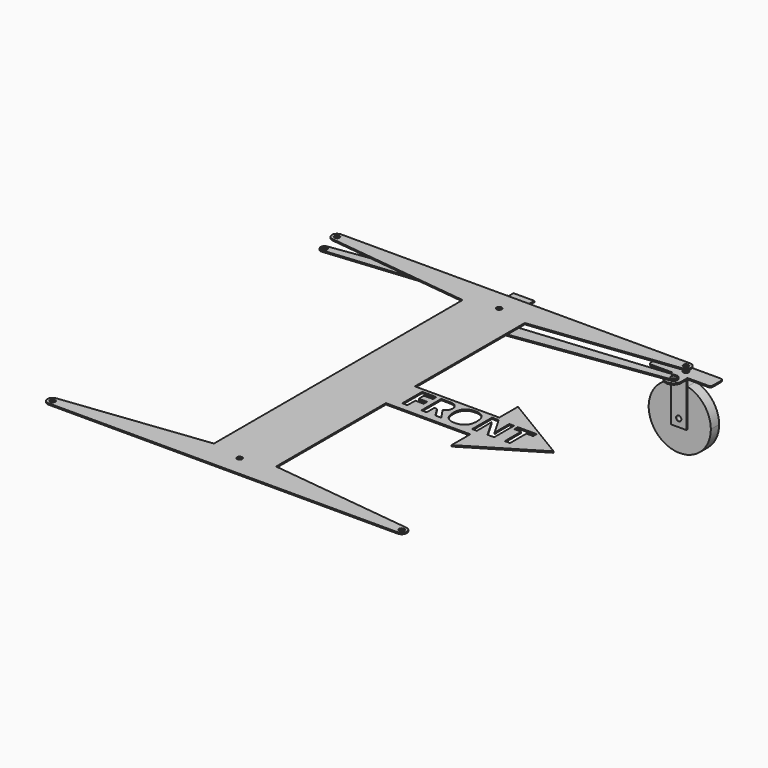
from build123d import *

# Parameters (mm, degrees)
F0_R      = 6.35
F1_DEPTH  = 3.175
F2_DEPTH  = 3.175
F3_R      = 6.35
F4_DEPTH  = 3.175
F6_R      = 6.35
F7_DEPTH  = 3.175
F8_R      = 6.35
F9_DEPTH  = 3.175
F10_DEPTH = 25.4


# Not quite as in the source:
# - a feature names something its author has since deleted; it is built from what else it names


with BuildPart() as f1:
    # F0 (on Top) → F1 (new body)
    with BuildSketch(Plane.XY):
        with BuildLine():
            Line((25.4, -29.2133073411), (25.4, 76.2))
            Line((25.4, 76.2), (-25.4, 76.2))
            Line((-25.4, 76.2), (-25.4, 66.4512439966))
            Line((-25.4, 66.4512439966), (-2.6644509402, 69.6627463851))
            ThreePointArc((-2.6644509402, 69.6627463851), (18.9170531521, 53.046686458), (1.8278232406, 31.8378914094))
            Line((1.8278232406, 31.8378914094), (-25.4, 29.2133073411))
            Line((-25.4, 29.2133073411), (-25.4, -76.2))
            Line((-25.4, -76.2), (25.4, -76.2))
            Line((25.4, -76.2), (25.4, -66.4512439966))
            Line((25.4, -66.4512439966), (2.6644509402, -69.6627463851))
            ThreePointArc((2.6644509402, -69.6627463851), (-18.9170531521, -53.046686458), (-1.8278232406, -31.8378914094))
            Line((-1.8278232406, -31.8378914094), (25.4, -29.2133073411))
        make_face()
        Circle(F0_R, mode=Mode.SUBTRACT)
        with BuildLine():
            Line((-2.6644509402, 69.6627463851), (-25.4, 66.4512439966))
            Line((-25.4, 66.4512439966), (-25.4, 29.2133073411))
            Line((-25.4, 29.2133073411), (1.8278232406, 31.8378914094))
            ThreePointArc((1.8278232406, 31.8378914094), (18.9170531521, 53.046686458), (-2.6644509402, 69.6627463851))
        make_face()
        with Locations((0, 50.8)):
            Circle(F0_R, mode=Mode.SUBTRACT)
        with BuildLine():
            Line((25.4, -66.4512439966), (25.4, -29.2133073411))
            Line((25.4, -29.2133073411), (-1.8278232406, -31.8378914094))
            ThreePointArc((-1.8278232406, -31.8378914094), (-18.9170531521, -53.046686458), (2.6644509402, -69.6627463851))
            Line((2.6644509402, -69.6627463851), (25.4, -66.4512439966))
        make_face()
        with Locations((0, -50.8)):
            Circle(F0_R, mode=Mode.SUBTRACT)
    extrude(amount=F1_DEPTH)


with BuildPart() as f2:
    # F0 (on Top) → F2 (new body)
    with BuildSketch(Plane.XY):
        with BuildLine():
            Line((426.8210296238, 9.4810542953), (25.4, -29.2133073411))
            Line((25.4, -29.2133073411), (25.4, -66.4512439966))
            Line((25.4, -66.4512439966), (429.0671667142, -9.4313731925))
            ThreePointArc((429.0671667142, -9.4313731925), (437.1934678202, 1.123343229), (426.8210296238, 9.4810542953))
        make_face()
        with Locations((427.7349412441, 0)):
            Circle(F0_R, mode=Mode.SUBTRACT)
        with BuildLine():
            Line((25.4, -66.4512439966), (25.4, -29.2133073411))
            Line((25.4, -29.2133073411), (-1.8278232406, -31.8378914094))
            ThreePointArc((-1.8278232406, -31.8378914094), (-18.9170531521, -53.046686458), (2.6644509402, -69.6627463851))
            Line((2.6644509402, -69.6627463851), (25.4, -66.4512439966))
        make_face()
        with Locations((0, -50.8)):
            Circle(F0_R, mode=Mode.SUBTRACT)
    extrude(amount=-F2_DEPTH)


with BuildPart() as f2b:
    # F0 (on Top) → F2, piece 2 (new body)
    with BuildSketch(Plane.XY):
        with BuildLine():
            Line((-25.4, 29.2133073411), (-25.4, 66.4512439966))
            Line((-25.4, 66.4512439966), (-429.0671667142, 9.4313731925))
            ThreePointArc((-429.0671667142, 9.4313731925), (-437.1934678202, -1.123343229), (-426.8210296239, -9.4810542953))
            Line((-426.8210296239, -9.4810542953), (-25.4, 29.2133073411))
        make_face()
        with Locations((-427.7349412441, 0)):
            Circle(F0_R, mode=Mode.SUBTRACT)
        with BuildLine():
            Line((-2.6644509402, 69.6627463851), (-25.4, 66.4512439966))
            Line((-25.4, 66.4512439966), (-25.4, 29.2133073411))
            Line((-25.4, 29.2133073411), (1.8278232406, 31.8378914094))
            ThreePointArc((1.8278232406, 31.8378914094), (18.9170531521, 53.046686458), (-2.6644509402, 69.6627463851))
        make_face()
        with Locations((0, 50.8)):
            Circle(F0_R, mode=Mode.SUBTRACT)
    extrude(amount=-F2_DEPTH)


with BuildPart() as f4:
    # F3 (on face) → F4 (new body)
    with BuildSketch(Plane(origin=(0, 0, -3.175), x_dir=(1, 0, 0), z_dir=(0, 0, -1))):
        with BuildLine():
            Line((446.7849412441, -19.05), (446.7849412441, 0))
            ThreePointArc((446.7849412441, 0), (433.9433178754, 18.009957235), (412.7315491596, 11.7388553939))
            Line((412.7315491596, 11.7388553939), (429.0671667142, 9.4313731925))
            ThreePointArc((429.0671667142, 9.4313731925), (437.1934678202, -1.123343229), (426.8210296238, -9.4810542953))
            Line((426.8210296238, -9.4810542953), (408.6849412441, -7.7328540002))
            Line((408.6849412441, -7.7328540002), (408.6849412441, -19.05))
            Line((408.6849412441, -19.05), (446.7849412441, -19.05))
        make_face()
        with BuildLine():
            Line((497.5849412441, -19.05), (446.7849412441, -19.05))
            Line((446.7849412441, -19.05), (446.7849412441, -38.1))
            ThreePointArc((446.7849412441, -38.1), (441.2053254257, -51.5703841816), (427.7349412441, -57.15))
            Line((427.7349412441, -57.15), (497.5849412441, -57.15))
            ThreePointArc((497.5849412441, -57.15), (502.0750693047, -55.2901280605), (503.9349412441, -50.8))
            Line((503.9349412441, -50.8), (503.9349412441, -25.4))
            ThreePointArc((503.9349412441, -25.4), (502.0750693047, -20.9098719395), (497.5849412441, -19.05))
        make_face()
        with BuildLine():
            Line((446.7849412441, -38.1), (446.7849412441, -19.05))
            Line((446.7849412441, -19.05), (408.6849412441, -19.05))
            Line((408.6849412441, -19.05), (408.6849412441, -38.1))
            ThreePointArc((408.6849412441, -38.1), (414.2645570625, -51.5703841816), (427.7349412441, -57.15))
            ThreePointArc((427.7349412441, -57.15), (441.2053254257, -51.5703841816), (446.7849412441, -38.1))
        make_face()
        with Locations((427.7349412441, -38.1)):
            Circle(F3_R, mode=Mode.SUBTRACT)
        with BuildLine():
            Line((429.0671667142, 9.4313731925), (412.7315491596, 11.7388553939))
            ThreePointArc((412.7315491596, 11.7388553939), (409.7249840092, 6.2083766312), (408.6849412441, 0))
            Line((408.6849412441, 0), (408.6849412441, -7.7328540002))
            Line((408.6849412441, -7.7328540002), (426.8210296238, -9.4810542953))
            ThreePointArc((426.8210296238, -9.4810542953), (437.1934678202, -1.123343229), (429.0671667142, 9.4313731925))
        make_face()
        with Locations((427.7349412441, 0)):
            Circle(F3_R, mode=Mode.SUBTRACT)
        with BuildLine():
            Line((408.6849412441, -38.1), (408.6849412441, -19.05))
            Line((408.6849412441, -19.05), (357.8849412441, -19.05))
            ThreePointArc((357.8849412441, -19.05), (353.3948131836, -20.9098719395), (351.5349412441, -25.4))
            Line((351.5349412441, -25.4), (351.5349412441, -50.8))
            ThreePointArc((351.5349412441, -50.8), (353.3948131836, -55.2901280605), (357.8849412441, -57.15))
            Line((357.8849412441, -57.15), (427.7349412441, -57.15))
            ThreePointArc((427.7349412441, -57.15), (414.2645570625, -51.5703841816), (408.6849412441, -38.1))
        make_face()
    extrude(amount=F4_DEPTH)

    # F8 (on face) → F9 (join)
    with BuildSketch(Plane.XZ.offset(-19.05)):
        with BuildLine():
            ThreePointArc((446.7849412441, -21.4696672547), (427.7349412441, -19.05), (408.6849412441, -21.4696672547))
            Line((408.6849412441, -21.4696672547), (408.6849412441, -114.3))
            Line((408.6849412441, -114.3), (446.7849412441, -114.3))
            Line((446.7849412441, -114.3), (446.7849412441, -21.4696672547))
        make_face()
        with Locations((427.7349412441, -95.25)):
            Circle(F8_R, mode=Mode.SUBTRACT)
        with BuildLine():
            Line((446.7849412441, -6.35), (408.6849412441, -6.35))
            Line((408.6849412441, -6.35), (408.6849412441, -21.4696672547))
            ThreePointArc((408.6849412441, -21.4696672547), (427.7349412441, -19.05), (446.7849412441, -21.4696672547))
            Line((446.7849412441, -21.4696672547), (446.7849412441, -6.35))
        make_face()
    extrude(amount=F9_DEPTH)


with BuildPart() as f7:
    # F6 (on offset) → F7 (new body)
    with BuildSketch(Plane.XY.offset(6.35)):
        with BuildLine():
            Line((-76.2, -16.5132760904), (76.2, -16.5132760904))
            Line((76.2, -16.5132760904), (429.2353362196, 25.4889407694))
            ThreePointArc((429.2353362196, 25.4889407694), (440.4126865529, 38.8515143949), (427.7349412441, 50.8))
            Line((427.7349412441, 50.8), (-427.7349412441, 50.8))
            ThreePointArc((-427.7349412441, 50.8), (-440.4126865529, 38.8515143949), (-429.2353362196, 25.4889407694))
            Line((-429.2353362196, 25.4889407694), (-76.2, -16.5132760904))
        make_face()
        with Locations((-427.7349412441, 38.1)):
            Circle(F6_R, mode=Mode.SUBTRACT)
        Circle(F6_R, mode=Mode.SUBTRACT)
        with Locations((427.7349412441, 38.1)):
            Circle(F6_R, mode=Mode.SUBTRACT)
        with BuildLine():
            Line((76.2, -16.5132760904), (3.000789951, -25.2221184612))
            ThreePointArc((3.000789951, -25.2221184612), (0, -25.4), (-3.000789951, -25.2221184612))
            Line((-3.000789951, -25.2221184612), (-76.2, -16.5132760904))
            Line((-76.2, -16.5132760904), (-76.2, -778.5132760904))
            Line((-76.2, -778.5132760904), (-3.000789951, -769.8044337197))
            ThreePointArc((-3.000789951, -769.8044337197), (0, -769.6265521808), (3.000789951, -769.8044337197))
            Line((3.000789951, -769.8044337197), (76.2, -778.5132760904))
            Line((76.2, -778.5132760904), (76.2, -441.9822692871))
            Line((76.2, -441.9822692871), (76.2, -353.0442828937))
            Line((76.2, -353.0442828937), (76.2, -16.5132760904))
        make_face()
        with BuildLine():
            ThreePointArc((-3.000789951, -25.2221184612), (0, -25.4), (3.000789951, -25.2221184612))
            Line((3.000789951, -25.2221184612), (76.2, -16.5132760904))
            Line((76.2, -16.5132760904), (-76.2, -16.5132760904))
            Line((-76.2, -16.5132760904), (-3.000789951, -25.2221184612))
        make_face()
        with BuildLine():
            Line((76.2, -778.5132760904), (-76.2, -778.5132760904))
            Line((-76.2, -778.5132760904), (-429.2353362196, -820.5154929502))
            ThreePointArc((-429.2353362196, -820.5154929502), (-440.4126865529, -833.8780665757), (-427.7349412441, -845.8265521808))
            Line((-427.7349412441, -845.8265521808), (427.7349412441, -845.8265521808))
            ThreePointArc((427.7349412441, -845.8265521808), (440.4126865529, -833.8780665757), (429.2353362196, -820.5154929502))
            Line((429.2353362196, -820.5154929502), (76.2, -778.5132760904))
        make_face()
        with Locations((-427.7349412441, -833.1265521808)):
            Circle(F6_R, mode=Mode.SUBTRACT)
        with Locations((0, -795.0265521808)):
            Circle(F6_R, mode=Mode.SUBTRACT)
        with Locations((427.7349412441, -833.1265521808)):
            Circle(F6_R, mode=Mode.SUBTRACT)
        with BuildLine():
            Line((-3.000789951, -769.8044337197), (-76.2, -778.5132760904))
            Line((-76.2, -778.5132760904), (76.2, -778.5132760904))
            Line((76.2, -778.5132760904), (3.000789951, -769.8044337197))
            ThreePointArc((3.000789951, -769.8044337197), (0, -769.6265521808), (-3.000789951, -769.8044337197))
        make_face()
        Polygon((283.0087542534, -353.0442828937), (76.2, -353.0442828937), (76.2, -441.9822692871), (283.0087542534, -441.9822692871), (283.0087542534, -422.9342937469), (272.2444606479, -422.9342937469), (272.2444606479, -361.9758875575), (283.0087542534, -361.9758875575), align=None)
        Polygon((113.757941251, -398.8391128369), (113.757941251, -422.9342937469), (101.0432638383, -422.9342937469), (101.0432638383, -361.9758875575), (135.9852786797, -361.9758875575), (135.9852786797, -372.5692284449), (113.757941251, -372.5692284449), (113.757941251, -388.2857971669), (134.4376369379, -388.2857971669), (134.4376369379, -398.8391128369), align=None, mode=Mode.SUBTRACT)
        with BuildLine():
            Line((167.7119343852, -399.546225012), (160.8409387215, -399.546225012))
            Line((160.8409387215, -399.546225012), (160.8409387215, -422.9342937469))
            Line((160.8409387215, -422.9342937469), (147.9127934823, -422.9342937469))
            Line((147.9127934823, -422.9342937469), (147.9127934823, -361.9758875575))
            Line((147.9127934823, -361.9758875575), (165.6706482948, -361.9758875575))
            add(Edge.make_bspline(
                [(165.6706482948, -361.9758875575), (178.1051491853, -361.9758875575), (184.062235717, -366.4987371303)],
                knots=[0, 0, 0, 1, 1, 1], degree=2))
            add(Edge.make_bspline(
                [(184.062235717, -366.4987371303), (190.0193222488, -371.0215867031), (190.0193222488, -380.2407284578)],
                knots=[0, 0, 0, 1, 1, 1], degree=2))
            add(Edge.make_bspline(
                [(190.0193222488, -380.2407284578), (190.0193222488, -385.6174493364), (187.0641270264, -389.8067554304)],
                knots=[0, 0, 0, 1, 1, 1], degree=2))
            add(Edge.make_bspline(
                [(187.0641270264, -389.8067554304), (184.1089318041, -393.9960615244), (178.6788439689, -396.3708910936)],
                knots=[0, 0, 0, 1, 1, 1], degree=2))
            add(Edge.make_bspline(
                [(178.6788439689, -396.3708910936), (192.4475187746, -416.9305111282), (196.6101413903, -422.9342937469)],
                knots=[0, 0, 0, 1, 1, 1], degree=2))
            Line((196.6101413903, -422.9342937469), (182.267771801, -422.9342937469))
            Line((182.267771801, -422.9342937469), (167.7119343852, -399.546225012))
        make_face(mode=Mode.SUBTRACT)
        with BuildLine():
            add(Edge.make_bspline(
                [(252.1651432229, -369.1070471347), (259.6098336702, -377.1988119309), (259.6098336702, -392.3683693477)],
                knots=[0, 0, 0, 1, 1, 1], degree=2))
            add(Edge.make_bspline(
                [(259.6098336702, -392.3683693477), (259.6098336702, -407.5112432862), (252.1051053967, -415.6430332999)],
                knots=[0, 0, 0, 1, 1, 1], degree=2))
            add(Edge.make_bspline(
                [(252.1051053967, -415.6430332999), (244.6003771232, -423.7748233136), (230.5915510127, -423.7748233136)],
                knots=[0, 0, 0, 1, 1, 1], degree=2))
            add(Edge.make_bspline(
                [(230.5915510127, -423.7748233136), (216.5827249022, -423.7748233136), (209.0779966287, -415.6430332999)],
                knots=[0, 0, 0, 1, 1, 1], degree=2))
            add(Edge.make_bspline(
                [(209.0779966287, -415.6430332999), (201.5732683552, -407.5112432862), (201.5732683552, -392.2883189128)],
                knots=[0, 0, 0, 1, 1, 1], degree=2))
            add(Edge.make_bspline(
                [(201.5732683552, -392.2883189128), (201.5732683552, -377.0653945394), (209.0980092374, -369.0403384389)],
                knots=[0, 0, 0, 1, 1, 1], degree=2))
            add(Edge.make_bspline(
                [(209.0980092374, -369.0403384389), (216.6227501196, -361.0152823385), (230.6716014476, -361.0152823385)],
                knots=[0, 0, 0, 1, 1, 1], degree=2))
            add(Edge.make_bspline(
                [(230.6716014476, -361.0152823385), (244.7204527756, -361.0152823385), (252.1651432229, -369.1070471347)],
                knots=[0, 0, 0, 1, 1, 1], degree=2))
        make_face(mode=Mode.SUBTRACT)
        with BuildLine():
            Line((283.0087542534, -295.8072240158), (283.0087542534, -353.0442828937))
            Line((283.0087542534, -353.0442828937), (283.0087542534, -361.9758875575))
            Line((283.0087542534, -361.9758875575), (288.5480658927, -361.9758875575))
            Line((288.5480658927, -361.9758875575), (315.018076372, -407.6313189386))
            Line((315.018076372, -407.6313189386), (315.3115946334, -407.6313189386))
            add(Edge.make_bspline(
                [(315.3115946334, -407.6313189386), (314.6845328932, -395.7438293534), (314.6845328932, -390.8340693451)],
                knots=[0, 0, 0, 1, 1, 1], degree=2))
            Line((314.6845328932, -390.8340693451), (314.6845328932, -361.9758875575))
            Line((314.6845328932, -361.9758875575), (326.3185294345, -361.9758875575))
            Line((326.3185294345, -361.9758875575), (326.3185294345, -422.9342937469))
            Line((326.3185294345, -422.9342937469), (309.8948485373, -422.9342937469))
            Line((309.8948485373, -422.9342937469), (283.3714711014, -376.8252432346))
            Line((283.3714711014, -376.8252432346), (283.0087542534, -376.8252432346))
            Line((283.0087542534, -376.8252432346), (283.0087542534, -376.9909752264))
            add(Edge.make_bspline(
                [(283.0087542534, -376.9909752264), (283.7984067543, -389.0684141514), (283.7984067543, -394.2495545683)],
                knots=[0.0068012605, 0.0068012605, 0.0068012605, 1, 1, 1], degree=2))
            Line((283.7984067543, -394.2495545683), (283.7984067543, -422.9342937469))
            Line((283.7984067543, -422.9342937469), (283.0087542534, -422.9342937469))
            Line((283.0087542534, -422.9342937469), (283.0087542534, -441.9822692871))
            Line((283.0087542534, -441.9822692871), (283.0087542534, -499.2193281651))
            Line((283.0087542534, -499.2193281651), (451.8381953239, -397.5132760904))
            Line((451.8381953239, -397.5132760904), (283.0087542534, -295.8072240158))
        make_face()
        Polygon((365.1830155868, -372.7293293147), (365.1830155868, -422.9342937469), (352.2548703477, -422.9342937469), (352.2548703477, -372.7293293147), (335.697772059, -372.7293293147), (335.697772059, -361.9758875575), (381.7267721364, -361.9758875575), (381.7267721364, -372.7293293147), align=None, mode=Mode.SUBTRACT)
    extrude(amount=F7_DEPTH)


with BuildPart() as f10:
    # F8 (on face) → F10 (new body)
    with BuildSketch(Plane.XZ.offset(-19.05)):
        with BuildLine():
            Line((408.6849412441, -114.3), (408.6849412441, -21.4696672547))
            ThreePointArc((408.6849412441, -21.4696672547), (381.0721616441, -155.4913894262), (503.9349412441, -95.25))
            ThreePointArc((503.9349412441, -95.25), (487.9763306703, -48.5872204), (446.7849412441, -21.4696672547))
            Line((446.7849412441, -21.4696672547), (446.7849412441, -114.3))
            Line((446.7849412441, -114.3), (408.6849412441, -114.3))
        make_face()
        with BuildLine():
            ThreePointArc((446.7849412441, -21.4696672547), (427.7349412441, -19.05), (408.6849412441, -21.4696672547))
            Line((408.6849412441, -21.4696672547), (408.6849412441, -114.3))
            Line((408.6849412441, -114.3), (446.7849412441, -114.3))
            Line((446.7849412441, -114.3), (446.7849412441, -21.4696672547))
        make_face()
        with Locations((427.7349412441, -95.25)):
            Circle(F8_R, mode=Mode.SUBTRACT)
    extrude(amount=-F10_DEPTH)


solid = Compound([f1.part, f2.part, f2b.part, f4.part, f7.part, f10.part])
